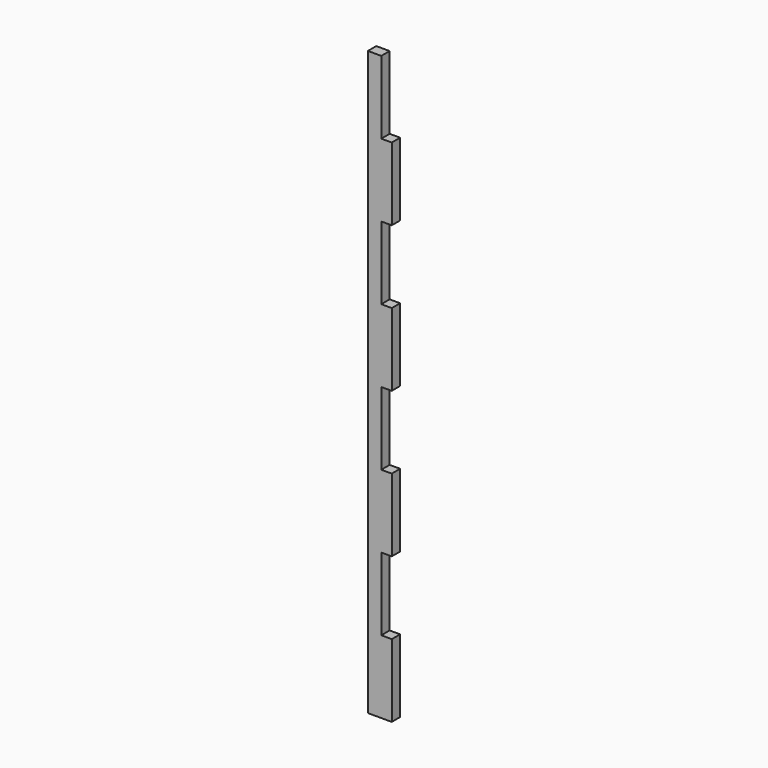
from build123d import *

# Parameters (mm, degrees)
F1_DEPTH = 18


# Not quite as in the source:
# - a feature names something its author has since deleted; it is built from what else it names


with BuildPart() as f1:
    # F0 (on Front) → F1 (new body)
    with BuildSketch(Plane.XZ):
        Polygon((0, 1000), (0, 0), (41, 0), (41, 125), (23, 125), (23, 250), (41, 250), (41, 375), (23, 375), (23, 500), (41, 500), (41, 625), (23, 625), (23, 750), (41, 750), (41, 875), (23, 875), (23, 1000), align=None)
    extrude(amount=F1_DEPTH)


solid = f1.part
